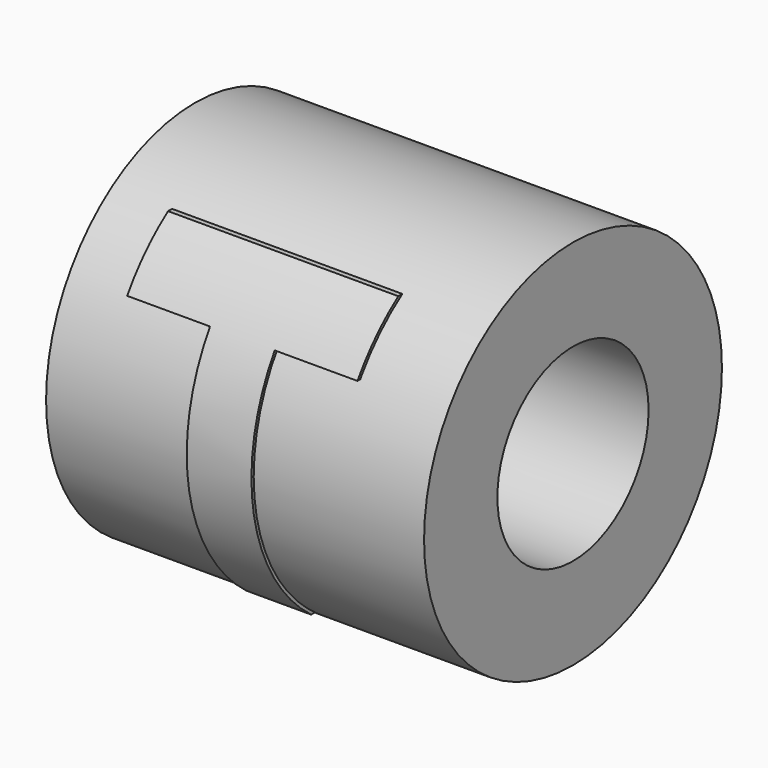
from build123d import *

# Parameters (mm, degrees)
F0_R         = 1
F0_R_2       = 0.985
F0_R_3       = 0.5
F1_DEPTH     = 2
F2_TEXT_SIZE = 2.2604994431
F3_REACH     = 3.0231687046
F4_DEPTH     = 2


# Not quite as in the source:
# - Text() gives the source's letters only with a copy of the font that has no kerning and outlines rounded to 1/6400 em; it was checked with that copy


with BuildPart() as f1:
    # F0 (on Right) → F1 (new body)
    with BuildSketch(Plane.YZ):
        Circle(F0_R)
        Circle(F0_R_2, mode=Mode.SUBTRACT)
        Circle(F0_R_2)
        Circle(F0_R_3, mode=Mode.SUBTRACT)
    extrude(amount=F1_DEPTH)

    f3_end = f1.faces().sort_by_distance((1, -1, 0))[0]
    # F2 (on Front) → F3 (intersect, up to a face of the model that its end follows)
    with BuildSketch(Plane.XZ):
        with Locations((0.2728080435, -0.7963191019)):
            Text('T', F2_TEXT_SIZE, font='Open Sans', font_style=FontStyle.BOLD, text_align=(TextAlign.LEFT, TextAlign.BOTTOM))
    f3_long = extrude(amount=F3_REACH, mode=Mode.PRIVATE)
    add(split(f3_long, bisect_by=f3_end, keep=Keep.BOTTOM, mode=Mode.PRIVATE), mode=Mode.INTERSECT)


with BuildPart() as f4:
    # F0 (on Right) → F4 (new body)
    with BuildSketch(Plane.YZ):
        Circle(F0_R_2)
        Circle(F0_R_3, mode=Mode.SUBTRACT)
    extrude(amount=F4_DEPTH)


solid = Compound([f1.part, f4.part])
